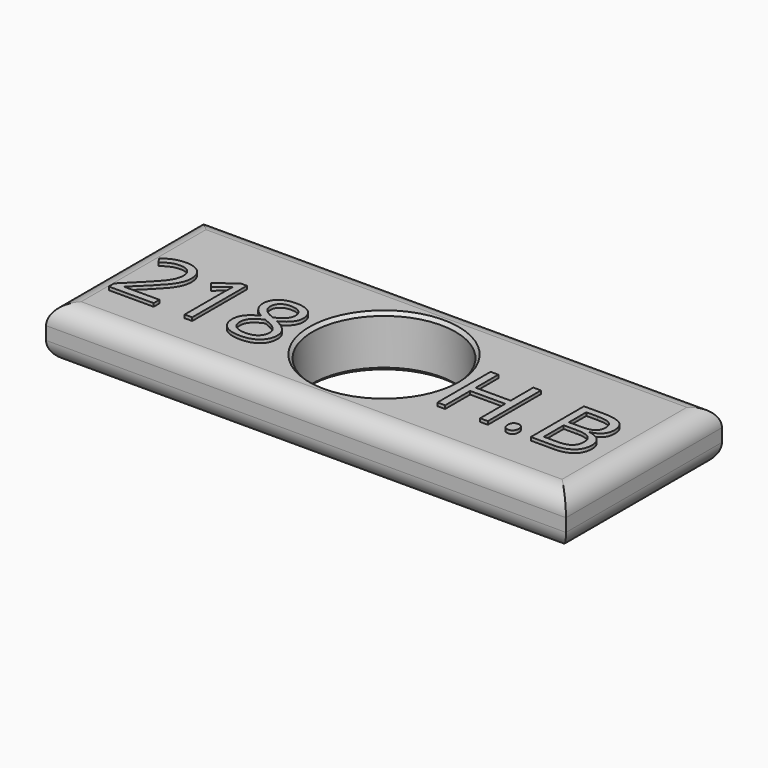
from build123d import *

# Parameters (mm, degrees)
F0_W         = 80
F0_H         = 30
F1_DEPTH     = 8
F2_R         = 11
F3_DEPTH     = 8.001
F4_R         = 3
F5_TEXT_SIZE = 14.7289787529
F6_DEPTH     = 0.5
F7_TEXT_SIZE = 14.3160740986
F8_DEPTH     = 0.5
F9_SIZE      = 0.5


# Not quite as in the source:
# - Text() gives the source's letters only with a copy of the font that has no kerning and outlines rounded to 1/6400 em; it was checked with that copy


with BuildPart() as f1:
    # F0 (on Top) → F1 (new body)
    with BuildSketch(Plane.XY):
        with Locations((2.7672089636, -12.8480492263)):
            Rectangle(F0_W, F0_H)
    extrude(amount=F1_DEPTH)

    # F2 (on face) → F3 (cut, through all)
    with BuildSketch(Plane.XY.offset(8)):
        with Locations((2.7672089636, -12.8480492263)):
            Circle(F2_R)
    extrude(amount=-F3_DEPTH, mode=Mode.SUBTRACT)

    # F4
    f4_edges = [f1.edges().sort_by_distance(p)[0] for p in [
        (2.767209, -27.848049, 8),
        (-37.232791, -12.848049, 8),
        (2.767209, 2.151951, 8),
        (42.767209, -12.848049, 8),
        (42.767209, -12.848049, 0),
        (2.767209, -27.848049, 0),
        (-37.232791, -12.848049, 0),
        (2.767209, 2.151951, 0),
    ]]
    fillet(f4_edges, radius=F4_R)

    # F5 (on face) → F6 (join)
    with BuildSketch(Plane.XY.offset(8)):
        with Locations((-34.2327910364, -20.4404944199)):
            Text('218', F5_TEXT_SIZE, font='Open Sans', text_align=(TextAlign.LEFT, TextAlign.BOTTOM))
    extrude(amount=F6_DEPTH)

    # F7 (on face) → F8 (join)
    with BuildSketch(Plane.XY.offset(8)):
        with Locations((14.7738168016, -19.3335196105)):
            Text('H.B', F7_TEXT_SIZE, font='Open Sans', text_align=(TextAlign.LEFT, TextAlign.BOTTOM))
    extrude(amount=F8_DEPTH)

    # F9
    f9_edges = [f1.edges().sort_by_distance(p)[0] for p in [
        (-8.232791, -12.848049, 8),
        (-8.232791, -12.848049, 0),
    ]]
    chamfer(f9_edges, length=F9_SIZE)


solid = f1.part
